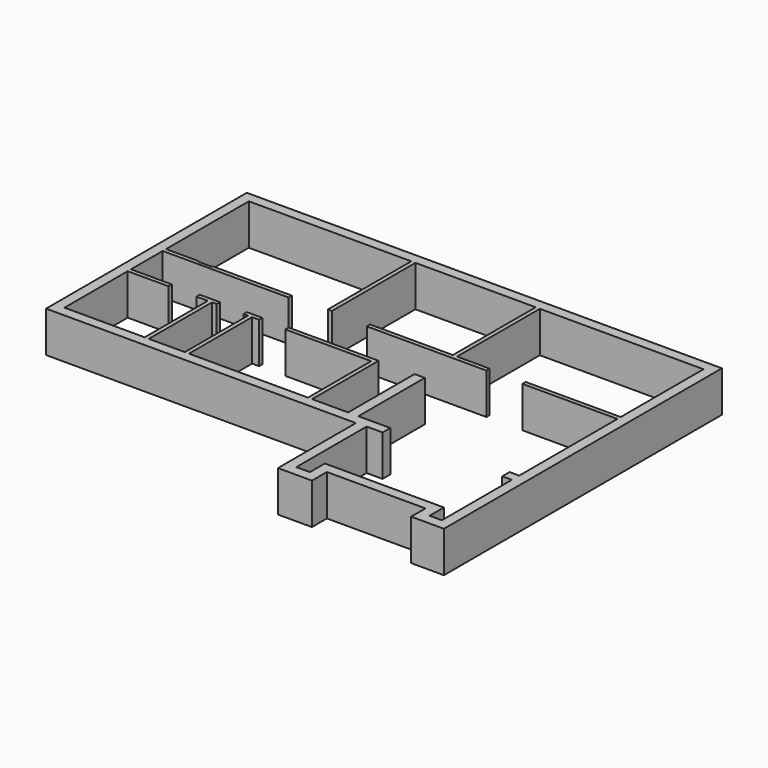
from build123d import *

# Parameters (mm, degrees)
F0_W     = 2.54
F0_H     = 64.262
F0_W_2   = 58.928
F0_H_2   = 2.54
F0_W_3   = 9.906
F0_H_3   = 5.969
F0_W_4   = 5.969
F0_H_4   = 5.715
F0_H_5   = 49.022
F0_W_5   = 25.3746
F1_DEPTH = 25.4


# Not quite as in the source:
# - a feature names something its author has since deleted; it is built from what else it names


with BuildPart() as f1:
    # F0 (on Top) → F1 (new body)
    with BuildSketch(Plane.XY):
        Polygon((-6.35, 73.152), (-6.35, -82.55), (185.928, -82.55), (185.928, -143.0351776838), (207.0404606759, -143.0351776838), (207.0404606759, -131.445), (268.2187365532, -131.445), (268.2187365532, -142.524239029), (288.544, -142.524239029), (288.544, -81.915), (288.544, 73.152), align=None)
        Polygon((0, 61.5773126483), (0, 66.802), (77.6735246181, 66.802), (100.838, 66.802), (103.378, 66.802), (178.054, 66.802), (180.594, 66.802), (282.194, 66.802), (282.194, 48.7640425563), (282.194, 2.54), (282.194, 0), (282.194, -64.607180655), (282.194, -76.2), (282.194, -81.915), (282.194, -136.174239029), (274.5687365532, -136.174239029), (274.5687365532, -125.095), (200.6904606759, -125.095), (200.6904606759, -136.6851776838), (192.278, -136.6851776838), (192.278, -82.169), (192.278, -76.2), (182.372, -76.2), (176.022, -76.2), (153.67, -76.2), (151.13, -76.2), (77.216, -76.2), (74.676, -76.2), (52.324, -76.2), (49.784, -76.2), (0, -76.2), (0, -27.178), (0, -24.638), (0, 0), (0, 2.54), (0, 17.2067563981), (0, 18.169073388), (0, 22.6956792176), align=None, mode=Mode.SUBTRACT)
        Polygon((18.6906643212, 2.54), (0, 2.54), (0, 0), (78.0796, 0), (78.0796, 2.54), (68.6789600206, 2.54), (68.1948126652, 2.54), (29.4852126652, 2.54), (29.2154226812, 2.54), (29.2154226812, 1.9534120802), (20.0714226812, 1.9534120802), (20.0714226812, 2.54), (19.6596, 2.54), align=None)
        Polygon((103.378, 66.802), (100.838, 66.802), (100.838, 48.322211951), (100.838, 2.0835588062), (103.378, 2.0835588062), align=None)
        Polygon((180.594, 2.54), (178.054, 2.54), (126.6382832546, 2.54), (126.6382832546, 0), (200.914, 0), (200.914, 2.54), (198.7368017435, 2.54), align=None)
        with Locations((179.324, 34.671)):
            Rectangle(F0_W, F0_H)
        with Locations((252.73, 1.27)):
            Rectangle(F0_W_2, F0_H_2)
        Polygon((176.022, -72.2413137555), (176.022, -76.2), (182.372, -76.2), (182.372, -66.0237371922), (182.372, -29.6653471887), (182.372, -24.638), (176.022, -24.638), (176.022, -31.1945881695), (176.022, -37.9491113126), (176.022, -44.4958023727), (176.022, -51.689), (176.022, -58.7322562933), (176.022, -65.4867812991), align=None)
        with Locations((197.231, -79.1845)):
            Rectangle(F0_W_3, F0_H_3)
        with Locations((279.2095, -79.0575)):
            Rectangle(F0_W_4, F0_H_4)
        Polygon((151.13, -64.7879913449), (151.13, -76.2), (153.67, -76.2), (153.67, -72.2413137555), (153.67, -65.4867812991), (153.67, -58.7322562933), (153.67, -51.689), (153.67, -46.2308526039), (153.67, -44.4958023727), (153.67, -37.9491113126), (153.67, -31.1945881695), (153.67, -27.178), (151.13, -27.178), (151.13, -46.2308526039), align=None)
        Polygon((97.8137195742, -27.178), (151.13, -27.178), (153.67, -27.178), (153.67, -24.638), (97.8137195742, -24.638), align=None)
        with Locations((75.946, -51.689)):
            Rectangle(F0_W, F0_H_5)
        Polygon((71.8879923224, -27.178), (74.676, -27.178), (77.216, -27.178), (81.5490037203, -27.178), (81.5490037203, -24.638), (71.8879923224, -24.638), align=None)
        with Locations((51.054, -51.689)):
            Rectangle(F0_W, F0_H_5)
        Polygon((42.6438264549, -27.178), (49.784, -27.178), (52.324, -27.178), (55.1770441234, -27.178), (55.1770441234, -24.638), (42.6438264549, -24.638), align=None)
        with Locations((12.6873, -25.908)):
            Rectangle(F0_W_5, F0_H_2)
    extrude(amount=F1_DEPTH)


solid = f1.part
